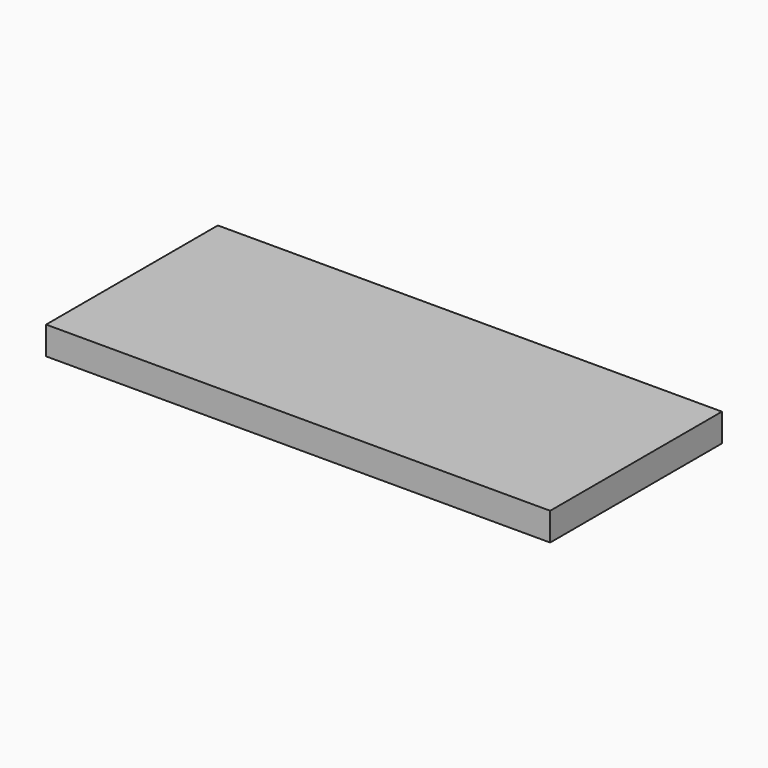
from build123d import *

# Parameters (mm, degrees)
F0_W     = 342.9
F0_H     = 146.05
F1_DEPTH = 19.05


# Not quite as in the source:
# - a length typed as a fraction of an inch, garbled in the dataset ("3 / 203.2 mm" for 3/8 in), is restored


with BuildPart() as f1:
    # F0 (on Top) → F1 (new body)
    with BuildSketch(Plane.XY):
        with Locations((9.2964811087, -92.757448221)):
            Rectangle(F0_W, F0_H)
    extrude(amount=F1_DEPTH)


solid = f1.part
